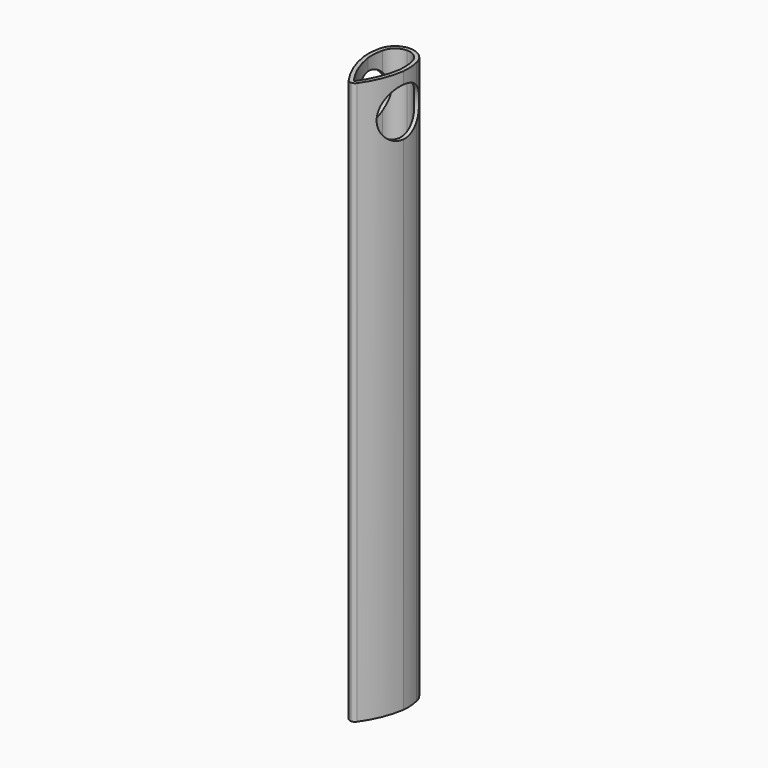
from build123d import *

# Parameters (mm, degrees)
F1_DEPTH = 50
F2_R     = 15.0073664172
F3_DEPTH = 25
F4_DEPTH = 300


# Not quite as in the source:
# - ends of sketch curves that miss each other by under 0.0002 mm in the source are joined


with BuildPart() as f1:
    # F0 (on Top) → F1 (new body)
    with BuildSketch(Plane.XY):
        with BuildLine():
            ThreePointArc((11.5946267397, 13.5320293348), (7.4846115717, 20.3323038327), (0, 22.9999896369))
            ThreePointArc((0, 22.9999896369), (-7.4846118013, 20.3323037509), (-11.5946270955, 13.5320290443))
            ThreePointArc((-11.5946270955, 13.5320290443), (-12.4147063987, 7.922168163), (-12.3388696742, 2.2531896672))
            ThreePointArc((-12.3388696742, 2.2531896672), (-8.8719983331, -10.2277960598), (-2.5843411657, -21.5529706895))
            ThreePointArc((-2.5843411657, -21.5529706895), (-1.4841666884, -22.619355112), (7e-08, -22.9998983316))
            ThreePointArc((7e-08, -22.9998983316), (1.4841670374, -22.6193504592), (2.5843454149, -21.5529672416))
            ThreePointArc((2.5843454149, -21.5529672416), (8.872000694, -10.2277939953), (12.3388707315, 2.2531898872))
            ThreePointArc((12.3388707315, 2.2531898872), (12.4147117976, 7.9221688824), (11.5946267397, 13.5320293348))
        make_face()
        with BuildLine():
            ThreePointArc((0, 20.5299898954), (5.9328912698, 18.410508519), (9.1798866708, 13.011580756))
            ThreePointArc((9.1798866708, 13.011580756), (9.9466025789, 7.8114966866), (9.8862458377, 2.5555396209))
            ThreePointArc((9.8862458377, 2.5555396209), (6.5447373666, -9.3927265107), (0.4963170659, -20.2252402669))
            ThreePointArc((0.4963170659, -20.2252402669), (0.2950851675, -20.4538524641), (4.0013e-05, -20.529391662))
            ThreePointArc((4.0013e-05, -20.529391662), (-0.2950640986, -20.4538699373), (-0.4963311707, -20.2252183832))
            ThreePointArc((-0.4963311707, -20.2252183832), (-6.5447290925, -9.3927429052), (-9.8862348466, 2.5554779538))
            ThreePointArc((-9.8862348466, 2.5554779538), (-9.9466064803, 7.8113582927), (-9.1799291893, 13.0113706774))
            ThreePointArc((-9.1799291893, 13.0113706774), (-5.9329742724, 18.4104406446), (0, 20.5299898954))
        make_face(mode=Mode.SUBTRACT)
    extrude(amount=F1_DEPTH)

    # F2 (on Right) → F3 (cut, symmetric)
    with BuildSketch(Plane.YZ):
        with Locations((2.2132990416, 27.6111345738)):
            Circle(F2_R)
    extrude(amount=F3_DEPTH, both=True, mode=Mode.SUBTRACT)

    # F4 (add): a face of the model
    f4_faces = [f1.faces().sort_by_distance(p)[0] for p in [
        (7.153517518, 19.9268403702, 0),
    ]]
    extrude(f4_faces, amount=F4_DEPTH)


solid = f1.part
